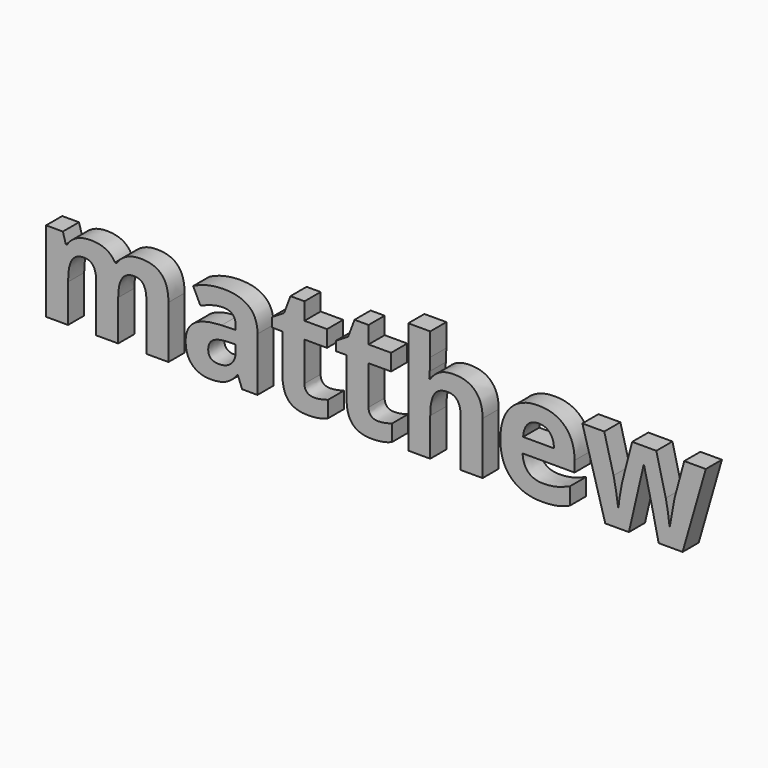
from build123d import *

# Parameters (mm, degrees)
F0_TEXT_SIZE = 185.9491018371
F1_DEPTH     = 25.4


# Not quite as in the source:
# - a feature of the source that left no trace in its solid (it failed there, or was rolled back) is left out
# - Text() gives the source's letters only with a copy of the font that has no kerning and outlines rounded to 1/6400 em; it was checked with that copy


with BuildPart() as f1:
    # F0 (on Front) → F1 (new body)
    with BuildSketch(Plane.XZ):
        with Locations((-107.7367663383, -47.7025024593)):
            Text('matthew', F0_TEXT_SIZE, font='Open Sans', font_style=FontStyle.BOLD, text_align=(TextAlign.LEFT, TextAlign.BOTTOM))
    extrude(amount=F1_DEPTH)


solid = f1.part
